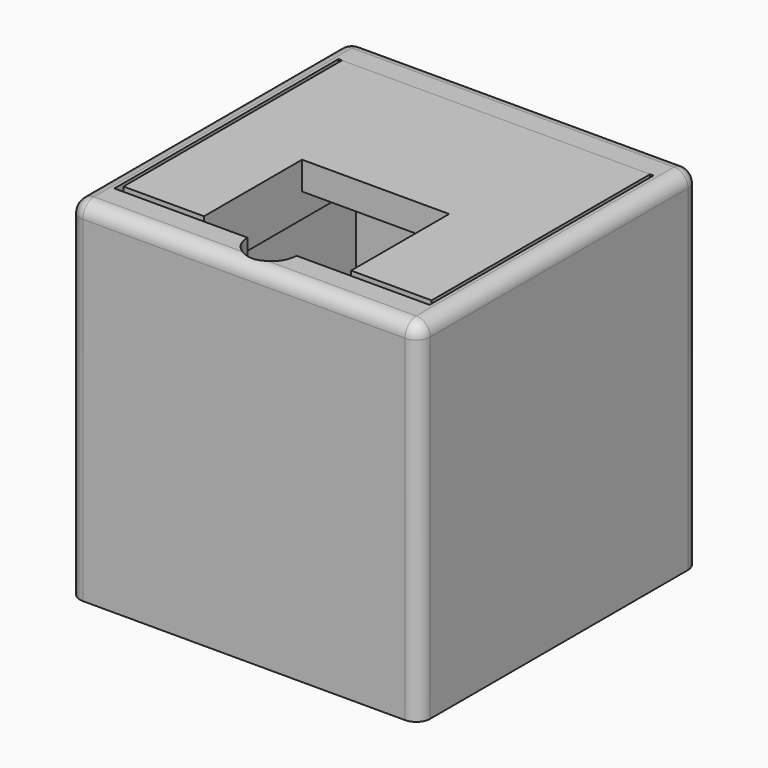
from build123d import *

# Parameters (mm, degrees)
F0_W          = 25.4
F0_H          = 25.4
F1_DEPTH      = 25.4
F0_W_2        = 1.27
F0_H_2        = 20.32
F0_W_3        = 20.32
F2_DEPTH      = 2.54
F3_DEPTH      = 21.59
F4_W          = 28.194
F4_H          = 28.194
F4_W_2        = 25.654
F4_H_2        = 25.654
F4_W_3        = 25.4
F4_H_3        = 25.4
F4_W_4        = 22.86
F4_H_4        = 20.32
F5_DEPTH      = 1.27
F6_DEPTH      = 2.54
F8_W          = 5.08
F8_H          = 0.635
F9_DEPTH      = 1.524
F10_W         = 12.7
F10_H         = 3.429
F11_DEPTH     = 2.286
F13_DEPTH     = 1.524
F14_DEPTH     = 1.27
F15_DEPTH     = 19.812
F8_W_2        = 10.668
F8_H_2        = 1.778
F16_DEPTH     = 1.016
F17_W         = 10.668
F17_H         = 8.89
F18_DEPTH     = 5.08
F19_C1_SIZE2  = 2.54
F19_C1_SIZE   = 3.81
F19_C2_SIZE2  = 2.54
F19_C2_SIZE   = 3.81
F20_T1_DEPTH  = 26.924
F20_T3_DEPTH  = 23.368
F20_T5_DEPTH  = 23.368
F20_S9_W      = 1.016
F20_S9_H      = 1.016
F20_T10_DEPTH = 1.016
F20_S15_W     = 1.016
F20_S15_H     = 1.016
F20_T16_DEPTH = 1.016
F20_S21_W     = 1.016
F20_S21_H     = 1.016
F20_T22_DEPTH = 1.016
F20_S27_W     = 1.016
F20_S27_H     = 1.016
F20_T28_DEPTH = 1.016


# Not quite as in the source:
# - a fillet or chamfer that OpenCascade refuses, or shapes differently, is made with other operations: its cross-section is extruded or revolved along the edge and cut away or added


with BuildPart() as f1:
    # F0 (on Top) → F1 (new body)
    with BuildSketch(Plane.XY):
        Rectangle(F0_W, F0_H)
        Polygon((10.16, 10.16), (11.43, 10.16), (11.43, -10.16), (10.16, -10.16), (-10.16, -10.16), (-11.43, -10.16), (-11.43, 10.16), (-10.16, 10.16), align=None, mode=Mode.SUBTRACT)
    extrude(amount=F1_DEPTH)

    # F0 (on Top) → F2 (join)
    with BuildSketch(Plane.XY):
        Rectangle(F0_W, F0_H)
        Polygon((10.16, 10.16), (11.43, 10.16), (11.43, -10.16), (10.16, -10.16), (-10.16, -10.16), (-11.43, -10.16), (-11.43, 10.16), (-10.16, 10.16), align=None, mode=Mode.SUBTRACT)
        with Locations((10.795, 0)):
            Rectangle(F0_W_2, F0_H_2)
        Rectangle(F0_W_3, F0_H_2)
        with Locations((-10.795, 0)):
            Rectangle(F0_W_2, F0_H_2)
    extrude(amount=F2_DEPTH)

    # F0 (on Top) → F3 (join)
    with BuildSketch(Plane.XY):
        with Locations((-10.795, 0)):
            Rectangle(F0_W_2, F0_H_2)
        with Locations((10.795, 0)):
            Rectangle(F0_W_2, F0_H_2)
    extrude(amount=F3_DEPTH)

    # F8 (on face) → F9 (cut)
    with BuildSketch(Plane.XZ.offset(-10.16)):
        with Locations((-6.35, 23.8125)):
            Rectangle(F8_W, F8_H)
        with Locations((-6.35, 24.4475)):
            Rectangle(F8_W, F8_H)
        with Locations((6.35, 23.8125)):
            Rectangle(F8_W, F8_H)
        with Locations((6.35, 24.4475)):
            Rectangle(F8_W, F8_H)
    extrude(amount=-F9_DEPTH, mode=Mode.SUBTRACT)

    # F10 (on face) → F11 (cut)
    with BuildSketch(Plane(origin=(0, -10.16, 0), x_dir=(-1, 0, 0), z_dir=(0, 1, 0))):
        with Locations((0, 21.3995)):
            Rectangle(F10_W, F10_H)
    extrude(amount=-F11_DEPTH, mode=Mode.SUBTRACT)

    # F12 (on face) → F13 (cut)
    with BuildSketch(Plane.XY.offset(25.4)):
        with BuildLine():
            Line((1.778, -10.16), (-1.778, -10.16))
            ThreePointArc((-1.778, -10.16), (0, -11.938), (1.778, -10.16))
        make_face()
    extrude(amount=-F13_DEPTH, mode=Mode.SUBTRACT)

    # F20: fillet of radius 1.016 on 8 edges, made by hand

    # F20_s2 → F20_t1 (cut)
    with BuildSketch(Plane.XY.offset(-2.54)):
        with BuildLine():
            ThreePointArc((12.7, -11.684), (12.4024204897, -12.4024204897), (11.684, -12.7))
            Line((11.684, -12.7), (12.7, -12.7))
            Line((12.7, -12.7), (12.7, -11.684))
        make_face()
        with BuildLine():
            ThreePointArc((-12.7, -11.684), (-12.4024204897, -12.4024204897), (-11.684, -12.7))
            Line((-11.684, -12.7), (-12.7, -12.7))
            Line((-12.7, -12.7), (-12.7, -11.684))
        make_face()
        with BuildLine():
            ThreePointArc((11.684, 12.7), (12.4024204897, 12.4024204897), (12.7, 11.684))
            Line((12.7, 11.684), (12.7, 12.7))
            Line((12.7, 12.7), (11.684, 12.7))
        make_face()
        with BuildLine():
            ThreePointArc((-11.684, 12.7), (-12.4024204897, 12.4024204897), (-12.7, 11.684))
            Line((-12.7, 11.684), (-12.7, 12.7))
            Line((-12.7, 12.7), (-11.684, 12.7))
        make_face()
    extrude(amount=F20_T1_DEPTH, mode=Mode.SUBTRACT)

    # F20_s4 → F20_t3 (cut)
    with BuildSketch(Plane.XZ.offset(-11.684)):
        with BuildLine():
            ThreePointArc((12.7, 24.384), (12.4024204897, 25.1024204897), (11.684, 25.4))
            Line((11.684, 25.4), (12.7, 25.4))
            Line((12.7, 25.4), (12.7, 24.384))
        make_face()
        with BuildLine():
            ThreePointArc((-11.684, 25.4), (-12.4024204897, 25.1024204897), (-12.7, 24.384))
            Line((-12.7, 24.384), (-12.7, 25.4))
            Line((-12.7, 25.4), (-11.684, 25.4))
        make_face()
    extrude(amount=F20_T3_DEPTH, mode=Mode.SUBTRACT)

    # F20_s6 → F20_t5 (cut)
    with BuildSketch(Plane.YZ.offset(-11.684)):
        with BuildLine():
            ThreePointArc((-11.684, 25.4), (-12.4024204897, 25.1024204897), (-12.7, 24.384))
            Line((-12.7, 24.384), (-12.7, 25.4))
            Line((-12.7, 25.4), (-11.684, 25.4))
        make_face()
        with BuildLine():
            ThreePointArc((12.7, 24.384), (12.4024204897, 25.1024204897), (11.684, 25.4))
            Line((11.684, 25.4), (12.7, 25.4))
            Line((12.7, 25.4), (12.7, 24.384))
        make_face()
    extrude(amount=F20_T5_DEPTH, mode=Mode.SUBTRACT)


with BuildPart() as f5:
    # F4 (on face) → F5 (new body)
    with BuildSketch(Plane.XY.offset(25.4)):
        Rectangle(F4_W, F4_H)
        Rectangle(F4_W_2, F4_H_2, mode=Mode.SUBTRACT)
        Rectangle(F4_W_2, F4_H_2)
        Rectangle(F4_W_3, F4_H_3, mode=Mode.SUBTRACT)
        Rectangle(F4_W_3, F4_H_3)
        Rectangle(F4_W_4, F4_H_4, mode=Mode.SUBTRACT)
        Rectangle(F4_W_4, F4_H_4)
    extrude(amount=F5_DEPTH)

    # F4 (on face) → F6 (join)
    with BuildSketch(Plane.XY.offset(25.4)):
        Rectangle(F4_W, F4_H)
        Rectangle(F4_W_2, F4_H_2, mode=Mode.SUBTRACT)
    extrude(amount=-F6_DEPTH)


with BuildPart() as f14:
    # F8 (on face) → F14 (new body)
    with BuildSketch(Plane.XZ.offset(-10.16)):
        with Locations((6.35, 24.4475)):
            Rectangle(F8_W, F8_H)
    extrude(amount=-F14_DEPTH)



with BuildPart() as f14b:
    # F8 (on face) → F14, piece 2 (new body)
    with BuildSketch(Plane.XZ.offset(-10.16)):
        with Locations((-6.35, 24.4475)):
            Rectangle(F8_W, F8_H)
    extrude(amount=-F14_DEPTH)


with BuildPart() as f14_1:
    add(f14.part)

    add(f14b.part)  # F15 merges F14b
    # F8 (on face) → F15 (join)
    with BuildSketch(Plane.XZ.offset(-10.16)):
        Polygon((-5.334, 23.368), (5.334, 23.368), (5.334, 21.59), (10.16, 21.59), (11.176, 21.59), (11.176, 25.4), (-11.176, 25.4), (-11.176, 21.59), (-10.16, 21.59), (-5.334, 21.59), align=None)
        Polygon((-8.89, 24.13), (-8.89, 24.765), (-3.81, 24.765), (-3.81, 24.13), (-3.81, 23.495), (-8.89, 23.495), align=None, mode=Mode.SUBTRACT)
        Polygon((3.81, 24.13), (3.81, 24.765), (8.89, 24.765), (8.89, 24.13), (8.89, 23.495), (3.81, 23.495), align=None, mode=Mode.SUBTRACT)
        with Locations((6.35, 24.4475)):
            Rectangle(F8_W, F8_H)
        with Locations((6.35, 23.8125)):
            Rectangle(F8_W, F8_H)
        with Locations((-6.35, 24.4475)):
            Rectangle(F8_W, F8_H)
        with Locations((-6.35, 23.8125)):
            Rectangle(F8_W, F8_H)
    extrude(amount=F15_DEPTH)

    # F8 (on face) → F16 (join)
    with BuildSketch(Plane.XZ.offset(-10.16)):
        with Locations((0, 22.479)):
            Rectangle(F8_W_2, F8_H_2)
    extrude(amount=F16_DEPTH)

    # F17 (on face) → F18 (cut)
    with BuildSketch(Plane.XY.offset(25.4)):
        with Locations((0, -5.207)):
            Rectangle(F17_W, F17_H)
    extrude(amount=-F18_DEPTH, mode=Mode.SUBTRACT)

    # F19: chamfer of 2.54 x 3.81 on 2 edges, made by hand

    # F19_c1
    f19_c1_edges = [f14_1.edges().sort_by_distance(p)[0] for p in [
        (8.255, -9.652, 21.59),
    ]]
    f19_c1_side = f14_1.faces().sort_by_distance((8.255, -9.6012, 21.59))[0]
    chamfer(f19_c1_edges, length=F19_C1_SIZE, length2=F19_C1_SIZE2, reference=f19_c1_side)

    # F19_c2
    f19_c2_edges = [f14_1.edges().sort_by_distance(p)[0] for p in [
        (-8.255, -9.652, 21.59),
    ]]
    f19_c2_side = f14_1.faces().sort_by_distance((-8.255, -9.6012, 21.59))[0]
    chamfer(f19_c2_edges, length=F19_C2_SIZE, length2=F19_C2_SIZE2, reference=f19_c2_side)


with BuildPart() as f20_tool8:
    # F20_s9 → F20_t10 (new body)
    with BuildSketch(Plane.YZ.offset(11.684)):
        with Locations((-12.192, 24.892)):
            Rectangle(F20_S9_W, F20_S9_H)
    extrude(amount=F20_T10_DEPTH)

    # F20_s11 → F20_t12 (revolve, cut)
    with BuildSketch(Plane(origin=(11.684, -11.684, 24.384), x_dir=(0, 0.7071067812, -0.7071067812), z_dir=(0, -0.7071067812, -0.7071067812))):
        with BuildLine():
            ThreePointArc((0, -1.016), (1.016, 0), (0, 1.016))
            Line((0, 1.016), (0, -1.016))
        make_face()
    revolve(axis=Axis((11.684, -11.684, 24.384), (1, 0, 0)), mode=Mode.SUBTRACT)


with BuildPart() as f1_1:
    add(f1.part)

    # F20_t7: cut F20_tool8
    add(f20_tool8.part, mode=Mode.SUBTRACT)


with BuildPart() as f20_tool14:
    # F20_s15 → F20_t16 (new body)
    with BuildSketch(Plane.XZ.offset(-11.684)):
        with Locations((12.192, 24.892)):
            Rectangle(F20_S15_W, F20_S15_H)
    extrude(amount=-F20_T16_DEPTH)

    # F20_s17 → F20_t18 (revolve, cut)
    with BuildSketch(Plane(origin=(11.684, 11.684, 24.384), x_dir=(-0.7071067812, 0, -0.7071067812), z_dir=(0.7071067812, 0, -0.7071067812))):
        with BuildLine():
            ThreePointArc((0, -1.016), (1.016, 0), (0, 1.016))
            Line((0, 1.016), (0, -1.016))
        make_face()
    revolve(axis=Axis((11.684, 11.684, 24.384), (0, 1, 0)), mode=Mode.SUBTRACT)


with BuildPart() as f1_2:
    add(f1_1.part)

    # F20_t13: cut F20_tool14
    add(f20_tool14.part, mode=Mode.SUBTRACT)


with BuildPart() as f20_tool20:
    # F20_s21 → F20_t22 (new body)
    with BuildSketch(Plane.XY.offset(24.384)):
        with Locations((-12.192, -12.192)):
            Rectangle(F20_S21_W, F20_S21_H)
    extrude(amount=F20_T22_DEPTH)

    # F20_s23 → F20_t24 (revolve, cut)
    with BuildSketch(Plane(origin=(-11.684, -11.684, 24.384), x_dir=(0.7071067812, 0.7071067812, 0), z_dir=(0.7071067812, -0.7071067812, 0))):
        with BuildLine():
            ThreePointArc((0, -1.016), (1.016, 0), (0, 1.016))
            Line((0, 1.016), (0, -1.016))
        make_face()
    revolve(axis=Axis((-11.684, -11.684, 24.384), (0, 0, 1)), mode=Mode.SUBTRACT)


with BuildPart() as f1_3:
    add(f1_2.part)

    # F20_t19: cut F20_tool20
    add(f20_tool20.part, mode=Mode.SUBTRACT)


with BuildPart() as f20_tool26:
    # F20_s27 → F20_t28 (new body)
    with BuildSketch(Plane.XZ.offset(-11.684)):
        with Locations((-12.192, 24.892)):
            Rectangle(F20_S27_W, F20_S27_H)
    extrude(amount=-F20_T28_DEPTH)

    # F20_s29 → F20_t30 (revolve, cut)
    with BuildSketch(Plane(origin=(-11.684, 11.684, 24.384), x_dir=(0.7071067812, 0, -0.7071067812), z_dir=(0.7071067812, 0, 0.7071067812))):
        with BuildLine():
            ThreePointArc((0, -1.016), (1.016, 0), (0, 1.016))
            Line((0, 1.016), (0, -1.016))
        make_face()
    revolve(axis=Axis((-11.684, 11.684, 24.384), (0, 1, 0)), mode=Mode.SUBTRACT)


with BuildPart() as f1_4:
    add(f1_3.part)

    # F20_t25: cut F20_tool26
    add(f20_tool26.part, mode=Mode.SUBTRACT)


solid = Compound([f14_1.part, f1_4.part])
